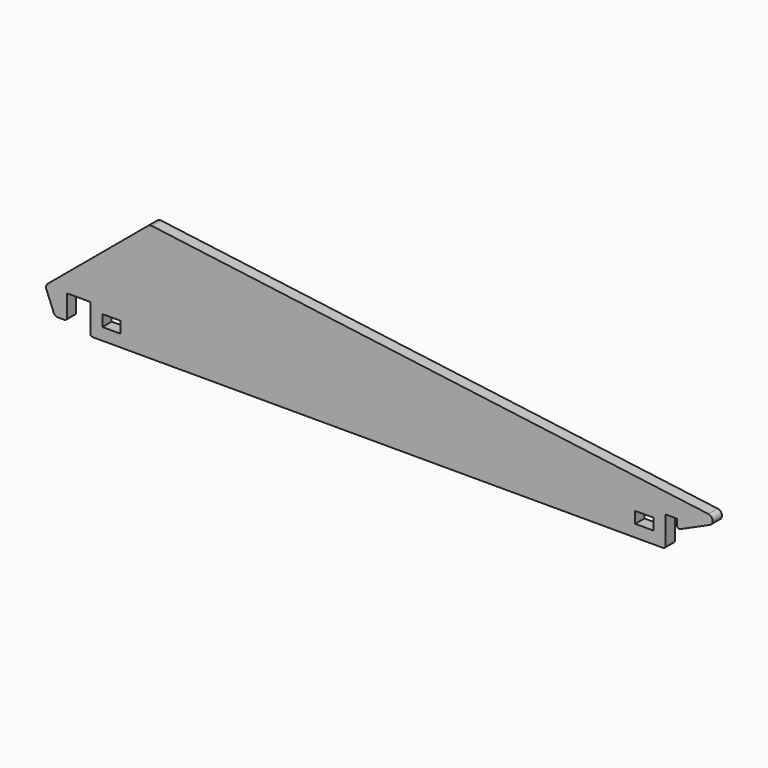
from build123d import *

# Parameters (mm, degrees)
F1_DEPTH = 6.096
F4_R     = 2.54
F5_R     = 1.27
F6_W     = 9.525
F6_H     = 5.969
F7_DEPTH = 6.097


# Not quite as in the source:
# - a feature of the source that left no trace in its solid (it failed there, or was rolled back) is left out


with BuildPart() as f1:
    # F0 (on Front) → F1 (new body)
    with BuildSketch(Plane.XZ):
        Polygon((-6.35, 0), (0, 0), (0, 12.7), (12.2428, 12.7), (12.2428, -3.175), (313.8678, -3.175), (313.8678, 12.7), (319.8368, 12.7), (319.8368, 7.62), (345.2368, 19.05), (43.434, 58.42), (0, 22.225), (-11.43, 12.7), align=None)
    extrude(amount=F1_DEPTH)

    # F4
    f4_edges = [f1.edges().sort_by_distance(p)[0] for p in [
        (43.434, -3.048, 58.42),
        (-11.43, -3.048, 12.7),
        (-6.35, -3.048, 0),
        (345.2368, -3.048, 19.05),
    ]]
    fillet(f4_edges, radius=F4_R)

    # F5
    f5_edges = [f1.edges().sort_by_distance(p)[0] for p in [
        (0, -3.048, 0),
        (12.2428, -3.048, -3.175),
        (319.8368, -3.048, 7.62),
        (313.8678, -3.048, -3.175),
    ]]
    fillet(f5_edges, radius=F5_R)

    # F6 (on face) → F7 (cut, through all)
    with BuildSketch(Plane.XZ.offset(6.096)):
        with Locations((23.3553, 6.1595)):
            Rectangle(F6_W, F6_H)
        with Locations((302.7553, 6.1595)):
            Rectangle(F6_W, F6_H)
    extrude(amount=-F7_DEPTH, mode=Mode.SUBTRACT)


solid = f1.part
